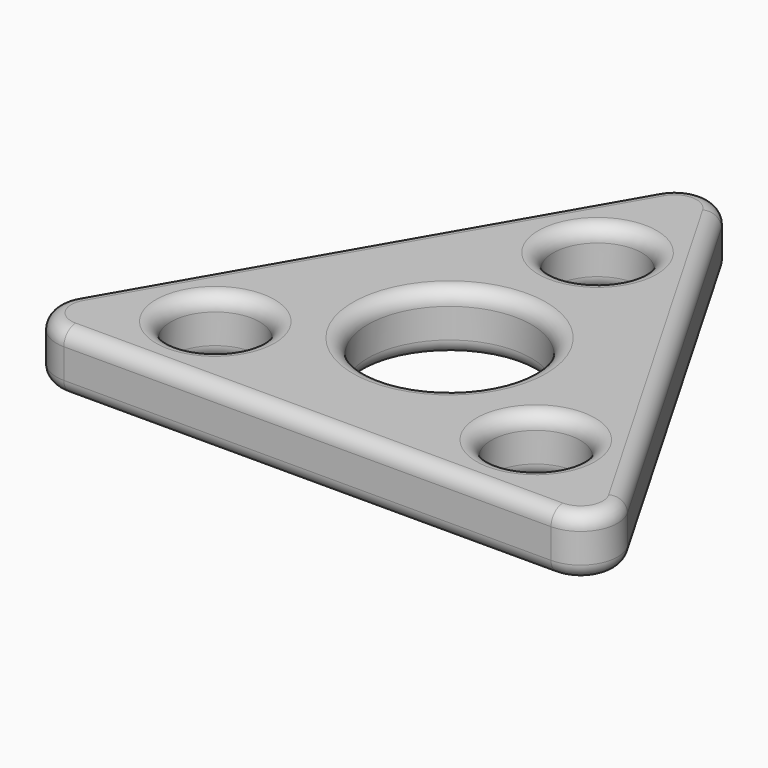
from build123d import *

# Parameters (mm, degrees)
F0_R         = 6
F0_R_2       = 11.05
F1_DEPTH     = 8
F2_R         = 2
F3_T1_DEPTH  = 8
F3_T4_ANGLE  = 120
F3_T6_ANGLE  = 120
F3_T8_ANGLE  = 120
F3_T10_ANGLE = 120
F3_T12_ANGLE = 120
F3_T14_ANGLE = 120


# Not quite as in the source:
# - a fillet or chamfer that OpenCascade refuses, or shapes differently, is made with other operations: its cross-section is extruded or revolved along the edge and cut away or added


with BuildPart() as f1:
    # F0 (on Top) → F1 (new body)
    with BuildSketch(Plane.XY):
        Polygon((-41.5692193817, -24), (41.5692193817, -24), (0, 48), align=None)
        with Locations((-21.6506350946, -12.5)):
            Circle(F0_R, mode=Mode.SUBTRACT)
        with Locations((21.6506350946, -12.5)):
            Circle(F0_R, mode=Mode.SUBTRACT)
        Circle(F0_R_2, mode=Mode.SUBTRACT)
        with Locations((0, 25)):
            Circle(F0_R, mode=Mode.SUBTRACT)
    extrude(amount=F1_DEPTH)

    # F2
    f2_edges = [f1.edges().sort_by_distance(p)[0] for p in [
        (0, -24, 8),
        (20.78461, 12, 8),
        (-20.78461, 12, 8),
        (-27.650635, -12.5, 8),
        (15.650635, -12.5, 8),
        (-11.05, 0, 8),
        (-6, 25, 8),
        (0, -24, 0),
        (20.78461, 12, 0),
        (-20.78461, 12, 0),
        (-27.650635, -12.5, 0),
        (15.650635, -12.5, 0),
        (-11.05, 0, 0),
        (-6, 25, 0),
    ]]
    fillet(f2_edges, radius=F2_R)

    # F3: fillet of radius 5 on 3 edges, made by hand

    # F3_s2 → F3_t1 (cut)
    with BuildSketch(Plane.XY):
        with BuildLine():
            ThreePointArc((32.9089653438, -24), (37.2390923627, -21.5), (37.2390923627, -16.5))
            Line((37.2390923627, -16.5), (41.5692193817, -24))
            Line((41.5692193817, -24), (32.9089653438, -24))
        make_face()
        with BuildLine():
            ThreePointArc((-32.9089653438, -24), (-37.2390923627, -21.5), (-37.2390923627, -16.5))
            Line((-37.2390923627, -16.5), (-41.5692193817, -24))
            Line((-41.5692193817, -24), (-32.9089653438, -24))
        make_face()
        with BuildLine():
            ThreePointArc((-4.3301270189, 40.5), (0, 43), (4.3301270189, 40.5))
            Line((4.3301270189, 40.5), (0, 48))
            Line((0, 48), (-4.3301270189, 40.5))
        make_face()
    extrude(amount=F3_T1_DEPTH, mode=Mode.SUBTRACT)

    # F3_s3 → F3_t4 (revolve, cut)
    with BuildSketch(Plane(origin=(16.4544826719, 28.5, 0), x_dir=(0, 0, 1), z_dir=(-0.5, -0.8660254038, 0))):
        with BuildLine():
            ThreePointArc((0, 22), (0.5857864376, 23.4142135624), (2, 24))
            Line((2, 24), (0, 24))
            Line((0, 24), (0, 22))
        make_face()
    revolve(axis=Axis((0, 38, 0), (0, 0, -1)), revolution_arc=F3_T4_ANGLE, mode=Mode.SUBTRACT)

    # F3_s5 → F3_t6 (revolve, cut)
    with BuildSketch(Plane(origin=(-16.4544826719, 28.5, 0), x_dir=(0, 0, 1), z_dir=(0.5, -0.8660254038, 0))):
        with BuildLine():
            ThreePointArc((8, -22), (7.4142135624, -23.4142135624), (6, -24))
            Line((6, -24), (8, -24))
            Line((8, -24), (8, -22))
        make_face()
    revolve(axis=Axis((0, 38, 8), (0, 0, 1)), revolution_arc=F3_T6_ANGLE, mode=Mode.SUBTRACT)

    # F3_s7 → F3_t8 (revolve, cut)
    with BuildSketch(Plane.YZ.offset(-32.9089653438)):
        with BuildLine():
            ThreePointArc((-22, 0), (-23.4142135624, 0.5857864376), (-24, 2))
            Line((-24, 2), (-24, 0))
            Line((-24, 0), (-22, 0))
        make_face()
    revolve(axis=Axis((-32.9089653438, -19, 0), (0, 0, -1)), revolution_arc=F3_T8_ANGLE, mode=Mode.SUBTRACT)

    # F3_s9 → F3_t10 (revolve, cut)
    with BuildSketch(Plane(origin=(-16.4544826719, -28.5, 0), x_dir=(0, 0, 1), z_dir=(0.5, 0.8660254038, 0))):
        with BuildLine():
            ThreePointArc((8, -22), (7.4142135624, -23.4142135624), (6, -24))
            Line((6, -24), (8, -24))
            Line((8, -24), (8, -22))
        make_face()
    revolve(axis=Axis((-32.9089653438, -19, 8), (0, 0, 1)), revolution_arc=F3_T10_ANGLE, mode=Mode.SUBTRACT)

    # F3_s11 → F3_t12 (revolve, cut)
    with BuildSketch(Plane(origin=(16.4544826719, -28.5, 0), x_dir=(0, 0, 1), z_dir=(-0.5, 0.8660254038, 0))):
        with BuildLine():
            ThreePointArc((0, 22), (0.5857864376, 23.4142135624), (2, 24))
            Line((2, 24), (0, 24))
            Line((0, 24), (0, 22))
        make_face()
    revolve(axis=Axis((32.9089653438, -19, 0), (0, 0, -1)), revolution_arc=F3_T12_ANGLE, mode=Mode.SUBTRACT)

    # F3_s13 → F3_t14 (revolve, cut)
    with BuildSketch(Plane.YZ.offset(32.9089653438)):
        with BuildLine():
            ThreePointArc((-22, 8), (-23.4142135624, 7.4142135624), (-24, 6))
            Line((-24, 6), (-24, 8))
            Line((-24, 8), (-22, 8))
        make_face()
    revolve(axis=Axis((32.9089653438, -19, 8), (0, 0, 1)), revolution_arc=F3_T14_ANGLE, mode=Mode.SUBTRACT)


solid = f1.part
